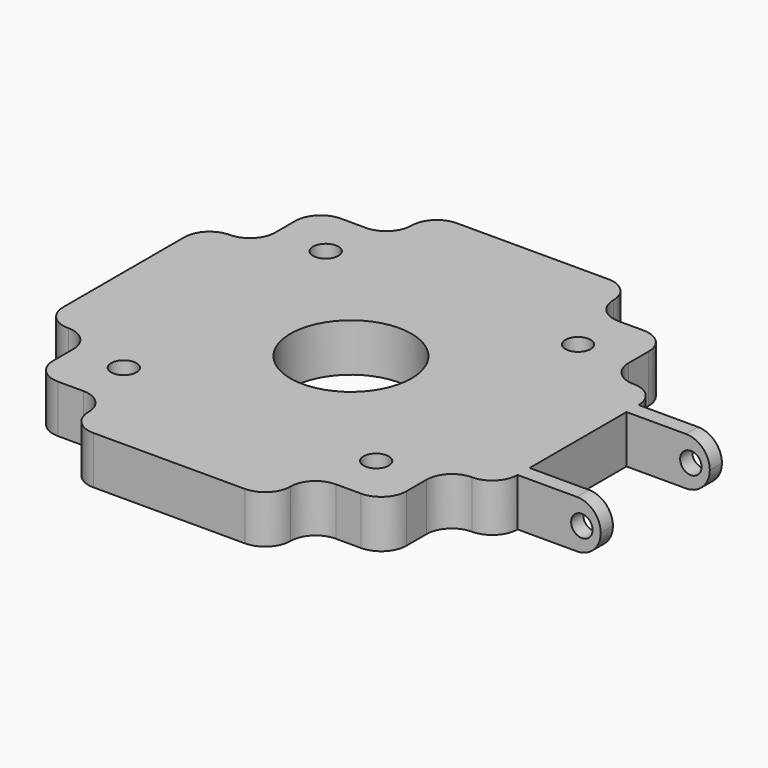
from build123d import *

# Parameters (mm, degrees)
F1_DEPTH  = 19
F2_R      = 24
F3_DEPTH  = 25
F4_R      = 9.99999
F5_R      = 5
F6_DEPTH  = 25
F7_R      = 7.5
F8_DEPTH  = 10
F9_W      = 6
F9_H      = 19
F10_DEPTH = 25
F11_DEPTH = 25
F12_R     = 4.25
F13_DEPTH = 250
F15_DEPTH = 8
F16_R     = 4.25
F17_DEPTH = 250
F18_R     = 9.49999


# Not quite as in the source:
# - a fillet or chamfer is up to 0.001 mm smaller than in the source, because OpenCascade refuses the exact size


with BuildPart() as f1:
    # F0 (on Top) → F1 (new body)
    with BuildSketch(Plane.XY):
        Polygon((0, 90), (-40, 90), (-40, 70), (-70, 70), (-70, 40), (-90, 40), (-90, 0), (0, 0), align=None)
        Polygon((40, 90), (0, 90), (0, 0), (90, 0), (90, 40), (70, 40), (70, 70), (40, 70), align=None)
        Polygon((0, -90), (0, 0), (-90, 0), (-90, -40), (-70, -40), (-70, -70), (-40, -70), (-40, -90), align=None)
        Polygon((90, 0), (0, 0), (0, -90), (40, -90), (40, -70), (70, -70), (70, -40), (90, -40), align=None)
    extrude(amount=F1_DEPTH)

    # F2 (on face) → F3 (cut)
    with BuildSketch(Plane.XY.offset(19)):
        Circle(F2_R)
    extrude(amount=-F3_DEPTH, mode=Mode.SUBTRACT)

    # F4 (radius 10 in the source; OpenCascade refuses exactly that, so slightly less here)
    f4_edges = [f1.edges().sort_by_distance(p)[0] for p in [
        (-70, 40, 9.5),
        (-40, 70, 9.5),
        (-40, 90, 9.5),
        (-70, 70, 9.5),
        (-90, 40, 9.5),
        (-40, -90, 9.5),
        (-40, -70, 9.5),
        (-70, -70, 9.5),
        (-70, -40, 9.5),
        (-90, -40, 9.5),
        (40, -90, 9.5),
        (40, -70, 9.5),
        (70, -70, 9.5),
        (70, -40, 9.5),
        (90, -40, 9.5),
        (90, 40, 9.5),
        (70, 40, 9.5),
        (70, 70, 9.5),
        (40, 70, 9.5),
        (40, 90, 9.5),
    ]]
    fillet(f4_edges, radius=F4_R)

    # F5 (on face) → F6 (cut)
    with BuildSketch(Plane.XY.offset(19)):
        with Locations((-50, -50)):
            Circle(F5_R)
        with Locations((50, -50)):
            Circle(F5_R)
        with Locations((-50, 50)):
            Circle(F5_R)
        with Locations((50, 50)):
            Circle(F5_R)
    extrude(amount=-F6_DEPTH, mode=Mode.SUBTRACT)

    # F7 (on face) → F8 (cut)
    with BuildSketch(Plane(origin=(0, 0, 0), x_dir=(1, 0, 0), z_dir=(0, 0, -1))):
        with Locations((-50, 50)):
            Circle(F7_R)
        with Locations((50, 50)):
            Circle(F7_R)
        with Locations((-50, -50)):
            Circle(F7_R)
        with Locations((50, -50)):
            Circle(F7_R)
    extrude(amount=-F8_DEPTH, mode=Mode.SUBTRACT)

    # F9 (on face) → F10 (join)
    with BuildSketch(Plane.YZ.offset(90)):
        with Locations((-27, 9.5)):
            Rectangle(F9_W, F9_H)
        with Locations((27, 9.5)):
            Rectangle(F9_W, F9_H)
    extrude(amount=F10_DEPTH)

    # F9 (on face) → F11 (join)
    with BuildSketch(Plane.YZ.offset(90)):
        with Locations((-27, 9.5)):
            Rectangle(F9_W, F9_H)
        with Locations((27, 9.5)):
            Rectangle(F9_W, F9_H)
    extrude(amount=F11_DEPTH)

    # F12 (on face) → F13 (cut)
    with BuildSketch(Plane.XZ.offset(30)):
        with BuildLine():
            ThreePointArc((125, 0), (134.5, 9.5), (125, 19))
            Line((125, 19), (115, 19))
            Line((115, 19), (115, 0))
            Line((115, 0), (125, 0))
        make_face()
        with Locations((125, 9.5)):
            Circle(F12_R, mode=Mode.SUBTRACT)
        with Locations((125, 9.5)):
            Circle(F12_R)
    extrude(amount=-F13_DEPTH, mode=Mode.SUBTRACT)

    # F15 (add): faces of the model
    f15_faces = [f1.faces().sort_by_distance(p)[0] for p in [
        (115, -27, 9.5),
        (115, 27, 9.5),
    ]]
    extrude(f15_faces, amount=F15_DEPTH)

    # F16 (on face) → F17 (cut)
    with BuildSketch(Plane.XZ.offset(30)):
        with Locations((115.5, 9.5)):
            Circle(F16_R)
    extrude(amount=-F17_DEPTH, mode=Mode.SUBTRACT)

    # F18 (radius 9.5 in the source; OpenCascade refuses exactly that, so slightly less here)
    f18_edges = [f1.edges().sort_by_distance(p)[0] for p in [
        (123, 27, 0),
        (123, -27, 0),
        (123, -27, 19),
        (123, 27, 19),
    ]]
    fillet(f18_edges, radius=F18_R)


solid = f1.part
